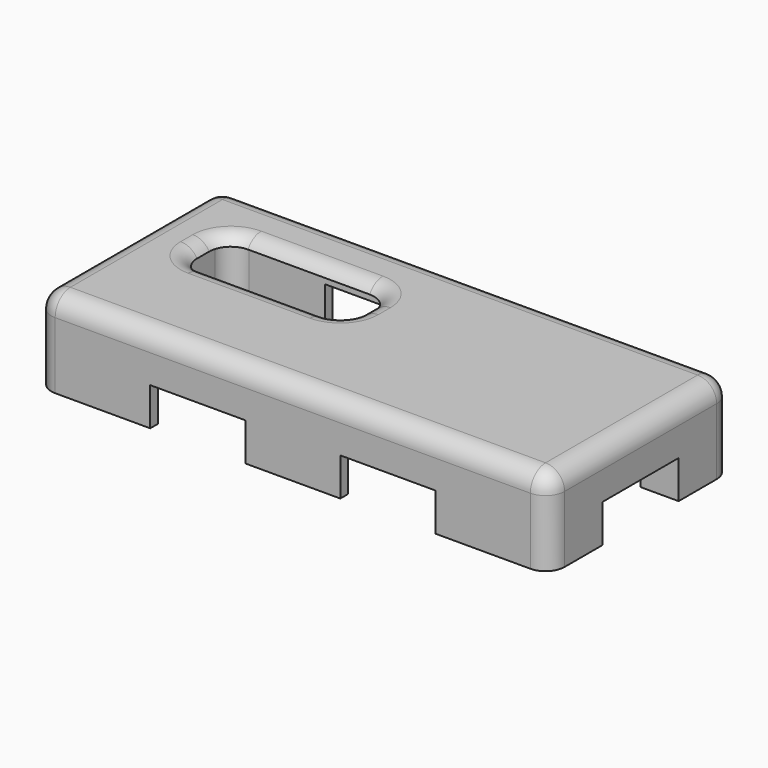
from build123d import *

# Parameters (mm, degrees)
F1_DEPTH     = 4.5
F2_R         = 1
F4_DEPTH     = 4
F5_W         = 12.5
F5_H         = 2.9783394848
F6_DEPTH     = 3.1
F7_T1_DEPTH  = 22
F7_T3_DEPTH  = 9
F7_T6_ANGLE  = 90
F7_T10_DEPTH = 22
F7_T16_DEPTH = 22
F7_T22_DEPTH = 22
F7_T26_ANGLE = 90
F7_T30_ANGLE = 90
F7_T36_ANGLE = 90
F7_T42_ANGLE = 90
F7_T46_ANGLE = 90
F8_W         = 1
F8_H         = 5
F8_W_2       = 2
F8_W_3       = 5
F8_H_2       = 0.5
F9_DEPTH     = 2


# Not quite as in the source:
# - a fillet or chamfer that OpenCascade refuses, or shapes differently, is made with other operations: its cross-section is extruded or revolved along the edge and cut away or added


with BuildPart() as f1:
    # F0 (on Top) → F1 (new body)
    with BuildSketch(Plane.XY):
        with BuildLine():
            ThreePointArc((0, 3.8761399509), (0.2928932188, 3.1690331698), (1, 2.8761399509))
            Line((1, 2.8761399509), (26, 2.8761399509))
            ThreePointArc((26, 2.8761399509), (26.7071067812, 3.1690331698), (27, 3.8761399509))
            Line((27, 3.8761399509), (27, 13.8761399509))
            ThreePointArc((27, 13.8761399509), (26.7071067812, 14.5832467321), (26, 14.8761399509))
            Line((26, 14.8761399509), (1, 14.8761399509))
            ThreePointArc((1, 14.8761399509), (0.2928932188, 14.5832467321), (0, 13.8761399509))
            Line((0, 13.8761399509), (0, 3.8761399509))
        make_face()
        with BuildLine():
            ThreePointArc((3, 10.6761399509), (3.2928932188, 11.3832467321), (4, 11.6761399509))
            Line((4, 11.6761399509), (10.4, 11.6761399509))
            ThreePointArc((10.4, 11.6761399509), (11.1071067812, 11.3832467321), (11.4, 10.6761399509))
            Line((11.4, 10.6761399509), (11.4, 9.8761399509))
            ThreePointArc((11.4, 9.8761399509), (11.1071067812, 9.1690331698), (10.4, 8.8761399509))
            Line((10.4, 8.8761399509), (4, 8.8761399509))
            ThreePointArc((4, 8.8761399509), (3.2928932188, 9.1690331698), (3, 9.8761399509))
            Line((3, 9.8761399509), (3, 10.6761399509))
        make_face(mode=Mode.SUBTRACT)
    extrude(amount=F1_DEPTH)

    # F2
    f2_edges = [f1.edges().sort_by_distance(p)[0] for p in [
        (0.292893, 3.169033, 4.5),
        (13.5, 2.87614, 4.5),
        (26.707107, 3.169033, 4.5),
        (27, 8.87614, 4.5),
        (26.707107, 14.583247, 4.5),
        (13.5, 14.87614, 4.5),
        (0.292893, 14.583247, 4.5),
        (0, 8.87614, 4.5),
        (3.292893, 11.383247, 4.5),
        (7.2, 11.67614, 4.5),
        (11.107107, 11.383247, 4.5),
        (11.4, 10.27614, 4.5),
        (11.107107, 9.169033, 4.5),
        (7.2, 8.87614, 4.5),
        (3.292893, 9.169033, 4.5),
        (3, 10.27614, 4.5),
    ]]
    fillet(f2_edges, radius=F2_R)

    # F3 (on Top) → F4 (cut)
    with BuildSketch(Plane.XY):
        with BuildLine():
            ThreePointArc((25, 13.3761399509), (24.7071067812, 14.0832467321), (24, 14.3761399509))
            Line((24, 14.3761399509), (2, 14.3761399509))
            ThreePointArc((2, 14.3761399509), (1.2928932188, 14.0832467321), (1, 13.3761399509))
            Line((1, 13.3761399509), (1, 4.3761399509))
            ThreePointArc((1, 4.3761399509), (1.2928932188, 3.6690331698), (2, 3.3761399509))
            Line((2, 3.3761399509), (14.5, 3.3761399509))
            Line((14.5, 3.3761399509), (24, 3.3761399509))
            ThreePointArc((24, 3.3761399509), (24.7071067812, 3.6690331698), (25, 4.3761399509))
            Line((25, 4.3761399509), (25, 13.3761399509))
        make_face()
    extrude(amount=F4_DEPTH, mode=Mode.SUBTRACT)

    # F5 (on Top) → F6 (cut)
    with BuildSketch(Plane.XY):
        with Locations((18.25, 14.7778680548)):
            Rectangle(F5_W, F5_H)
    extrude(amount=F6_DEPTH, mode=Mode.SUBTRACT)

    # F7: fillet of radius 1 on 8 edges, made by hand

    # F7_s2 → F7_t1 (join)
    with BuildSketch(Plane.YZ.offset(2)):
        with BuildLine():
            ThreePointArc((3.3761399509, 3), (3.6690331698, 3.7071067812), (4.3761399509, 4))
            Line((4.3761399509, 4), (3.3761399509, 4))
            Line((3.3761399509, 4), (3.3761399509, 3))
        make_face()
    extrude(amount=F7_T1_DEPTH)

    # F7_s4 → F7_t3 (join)
    with BuildSketch(Plane.XZ.offset(-13.3761399509)):
        with BuildLine():
            ThreePointArc((25, 3), (24.7071067812, 3.7071067812), (24, 4))
            Line((24, 4), (25, 4))
            Line((25, 4), (25, 3))
        make_face()
        with BuildLine():
            ThreePointArc((1, 3), (1.2928932188, 3.7071067812), (2, 4))
            Line((2, 4), (1, 4))
            Line((1, 4), (1, 3))
        make_face()
    extrude(amount=F7_T3_DEPTH)

    # F7_s5 → F7_t6 (revolve)
    with BuildSketch(Plane.XZ.offset(-4.3761399509)):
        with BuildLine():
            ThreePointArc((1, 3), (1.2928932188, 3.7071067812), (2, 4))
            Line((2, 4), (1, 4))
            Line((1, 4), (1, 3))
        make_face()
    revolve(axis=Axis((2, 4.3761399509, 4), (0, 0, 1)), revolution_arc=F7_T6_ANGLE)


with BuildPart() as f7_tool8:
    # F7_s9 → F7_t10 (new body)
    with BuildSketch(Plane.YZ.offset(24)):
        with BuildLine():
            ThreePointArc((14.3761399509, 3), (14.0832467321, 3.7071067812), (13.3761399509, 4))
            Line((13.3761399509, 4), (14.3761399509, 4))
            Line((14.3761399509, 4), (14.3761399509, 3))
        make_face()
    extrude(amount=-F7_T10_DEPTH)

    split(bisect_by=Plane.YZ.offset(12), keep=Keep.TOP)

    split(bisect_by=Plane.XY.offset(3.1), keep=Keep.TOP)


with BuildPart() as f1_1:
    add(f1.part)

    # F7_t7: union F7_tool8
    add(f7_tool8.part)


with BuildPart() as f7_tool14:
    # F7_s15 → F7_t16 (new body)
    with BuildSketch(Plane.YZ.offset(24)):
        with BuildLine():
            ThreePointArc((14.3761399509, 3), (14.0832467321, 3.7071067812), (13.3761399509, 4))
            Line((13.3761399509, 4), (14.3761399509, 4))
            Line((14.3761399509, 4), (14.3761399509, 3))
        make_face()
    extrude(amount=-F7_T16_DEPTH)

    split(bisect_by=Plane.YZ.offset(12), keep=Keep.BOTTOM)

    split(bisect_by=Plane.XY.offset(3.1), keep=Keep.BOTTOM)


with BuildPart() as f1_2:
    add(f1_1.part)

    # F7_t13: union F7_tool14
    add(f7_tool14.part)


with BuildPart() as f7_tool20:
    # F7_s21 → F7_t22 (new body)
    with BuildSketch(Plane.YZ.offset(24)):
        with BuildLine():
            ThreePointArc((14.3761399509, 3), (14.0832467321, 3.7071067812), (13.3761399509, 4))
            Line((13.3761399509, 4), (14.3761399509, 4))
            Line((14.3761399509, 4), (14.3761399509, 3))
        make_face()
    extrude(amount=-F7_T22_DEPTH)

    split(bisect_by=Plane.YZ.offset(12), keep=Keep.BOTTOM)

    split(bisect_by=Plane.XY.offset(3.1), keep=Keep.TOP)


with BuildPart() as f1_3:
    add(f1_2.part)

    # F7_t19: union F7_tool20
    add(f7_tool20.part)

    # F7_s25 → F7_t26 (revolve)
    with BuildSketch(Plane.YZ.offset(2)):
        with BuildLine():
            ThreePointArc((14.3761399509, 3), (14.0832467321, 3.7071067812), (13.3761399509, 4))
            Line((13.3761399509, 4), (14.3761399509, 4))
            Line((14.3761399509, 4), (14.3761399509, 3))
        make_face()
    revolve(axis=Axis((2, 13.3761399509, 4), (0, 0, 1)), revolution_arc=F7_T26_ANGLE)


with BuildPart() as f7_tool28:
    # F7_s29 → F7_t30 (revolve)
    with BuildSketch(Plane.XZ.offset(-13.3761399509)):
        with BuildLine():
            ThreePointArc((25, 3), (24.7071067812, 3.7071067812), (24, 4))
            Line((24, 4), (25, 4))
            Line((25, 4), (25, 3))
        make_face()
    revolve(axis=Axis((24, 13.3761399509, 4), (0, 0, 1)), revolution_arc=F7_T30_ANGLE)

    split(bisect_by=Plane.YZ.offset(24.5), keep=Keep.TOP)

    split(bisect_by=Plane.XY.offset(3.1), keep=Keep.BOTTOM)


with BuildPart() as f1_4:
    add(f1_3.part)

    # F7_t27: union F7_tool28
    add(f7_tool28.part)


with BuildPart() as f7_tool34:
    # F7_s35 → F7_t36 (revolve)
    with BuildSketch(Plane.XZ.offset(-13.3761399509)):
        with BuildLine():
            ThreePointArc((25, 3), (24.7071067812, 3.7071067812), (24, 4))
            Line((24, 4), (25, 4))
            Line((25, 4), (25, 3))
        make_face()
    revolve(axis=Axis((24, 13.3761399509, 4), (0, 0, 1)), revolution_arc=F7_T36_ANGLE)

    split(bisect_by=Plane.YZ.offset(24.5), keep=Keep.TOP)

    split(bisect_by=Plane.XY.offset(3.1), keep=Keep.TOP)


with BuildPart() as f1_5:
    add(f1_4.part)

    # F7_t33: union F7_tool34
    add(f7_tool34.part)


with BuildPart() as f7_tool40:
    # F7_s41 → F7_t42 (revolve)
    with BuildSketch(Plane.XZ.offset(-13.3761399509)):
        with BuildLine():
            ThreePointArc((25, 3), (24.7071067812, 3.7071067812), (24, 4))
            Line((24, 4), (25, 4))
            Line((25, 4), (25, 3))
        make_face()
    revolve(axis=Axis((24, 13.3761399509, 4), (0, 0, 1)), revolution_arc=F7_T42_ANGLE)

    split(bisect_by=Plane.YZ.offset(24.5), keep=Keep.BOTTOM)

    split(bisect_by=Plane.XY.offset(3.1), keep=Keep.TOP)


with BuildPart() as f1_6:
    add(f1_5.part)

    # F7_t39: union F7_tool40
    add(f7_tool40.part)

    # F7_s45 → F7_t46 (revolve)
    with BuildSketch(Plane.YZ.offset(24)):
        with BuildLine():
            ThreePointArc((3.3761399509, 3), (3.6690331698, 3.7071067812), (4.3761399509, 4))
            Line((4.3761399509, 4), (3.3761399509, 4))
            Line((3.3761399509, 4), (3.3761399509, 3))
        make_face()
    revolve(axis=Axis((24, 4.3761399509, 4), (0, 0, 1)), revolution_arc=F7_T46_ANGLE)

    # F8 (on face) → F9 (cut)
    with BuildSketch(Plane(origin=(0, 0, 0), x_dir=(1, 0, 0), z_dir=(0, 0, -1))):
        with Locations((0.5, -8.8761399509)):
            Rectangle(F8_W, F8_H)
        with Locations((26, -8.8761399509)):
            Rectangle(F8_W_2, F8_H)
        with Locations((8.5, -3.1261399509)):
            Rectangle(F8_W_3, F8_H_2)
        with Locations((18.5, -3.1261399509)):
            Rectangle(F8_W_3, F8_H_2)
        with Locations((8.5, -14.6261399509)):
            Rectangle(F8_W_3, F8_H_2)
    extrude(amount=-F9_DEPTH, mode=Mode.SUBTRACT)


solid = f1_6.part
